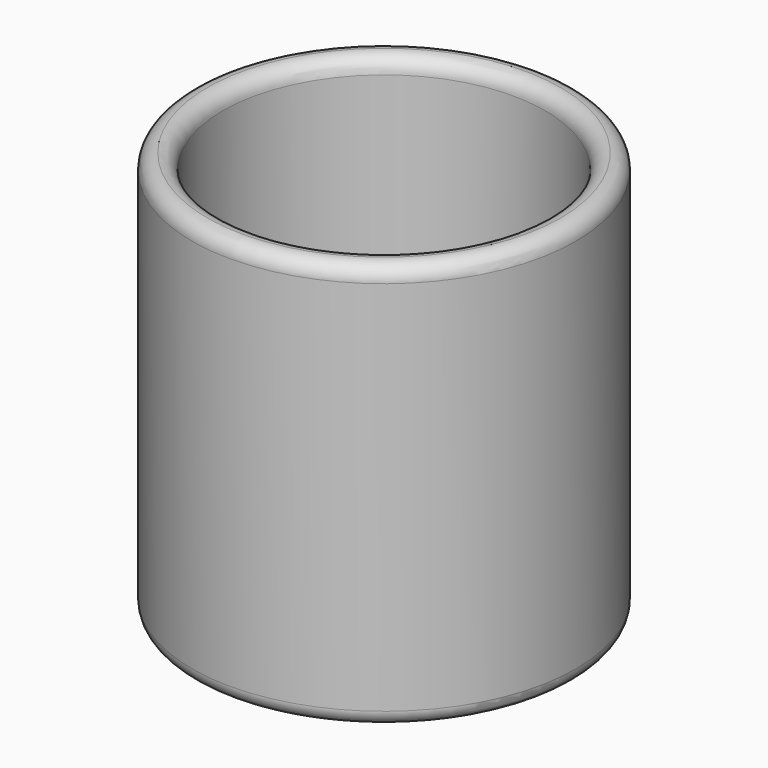
from build123d import *

# Parameters (mm, degrees)
F0_R     = 25
F1_DEPTH = 3
F2_R     = 25
F2_R_2   = 21
F3_DEPTH = 50
F4_R     = 1.99999


# Not quite as in the source:
# - a fillet or chamfer is up to 0.001 mm smaller than in the source, because OpenCascade refuses the exact size


with BuildPart() as f1:
    # F0 (on Top) → F1 (new body)
    with BuildSketch(Plane.XY):
        Circle(F0_R)
    extrude(amount=F1_DEPTH)

    # F2 (on face) → F3 (join)
    with BuildSketch(Plane.XY.offset(3)):
        Circle(F2_R)
        Circle(F2_R_2, mode=Mode.SUBTRACT)
    extrude(amount=F3_DEPTH)

    # F4 (radius 2 in the source; OpenCascade refuses exactly that, so slightly less here)
    f4_edges = [f1.edges().sort_by_distance(p)[0] for p in [
        (-25, 0, 53),
        (-21, 0, 53),
        (-21, 0, 3),
        (-25, 0, 0),
    ]]
    fillet(f4_edges, radius=F4_R)


solid = f1.part
